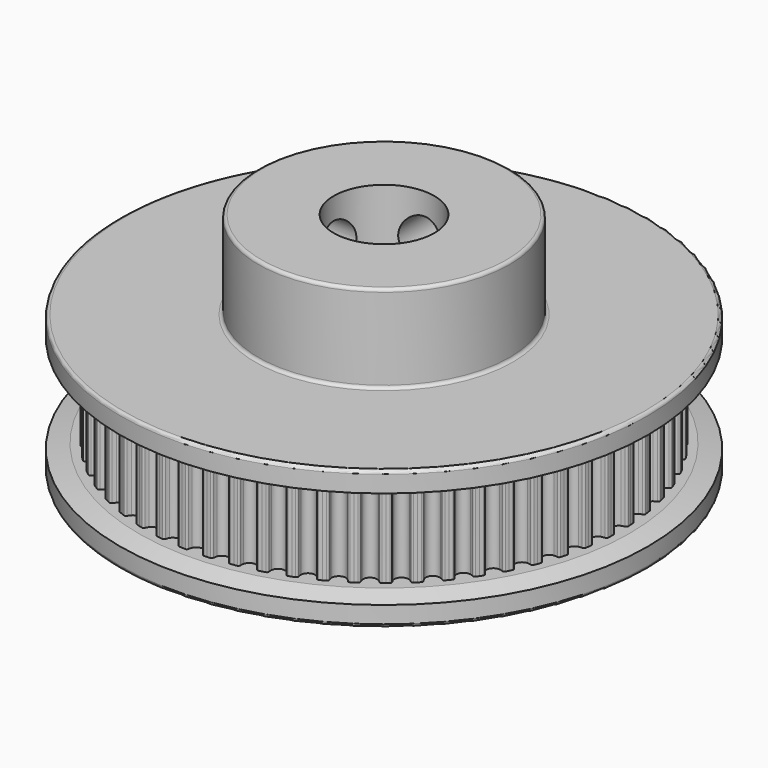
from build123d import *

# Parameters (mm, degrees)
F3_DEPTH    = 3.5
F4_COUNT    = 60
F5_R        = 21
F6_DEPTH    = 2
F7_R        = 21
F8_DEPTH    = 2
F9_R        = 10
F10_DEPTH   = 7
F11_R       = 4
F12_DEPTH   = 18.001
F13_R       = 1.75
F14_DEPTH   = 21.001
F15_R       = 1.75
F16_DEPTH   = 21.001
F17_SIZE2   = 0.4019237886
F17_SIZE    = 1.5
F17_2_SIZE2 = 0.4019237886
F17_2_SIZE  = 1.5
F18_R       = 0.25


# Not quite as in the source:
# - a feature names something its author has since deleted; it is built from what else it names


with BuildPart() as f3:
    # F2 (on Top) → F3 (new body, symmetric)
    with BuildSketch(Plane.XY):
        with BuildLine():
            ThreePointArc((0.5075672794, 18.4356928737), (0.3028425699, 18.1951004644), (0, 18.1051933345))
            ThreePointArc((0, 18.1051933345), (-0.3028425699, 18.1951004644), (-0.5075672794, 18.4356928737))
            ThreePointArc((-0.5075672794, 18.4356928737), (-0.5546426952, 18.5657821373), (-0.5833135378, 18.7011235355))
            ThreePointArc((-0.5833135378, 18.7011235355), (-0.6356764359, 18.7953689183), (-0.7377280214, 18.830147348))
            ThreePointArc((-0.7377280214, 18.830147348), (-0.8620076923, 18.8248674503), (-0.9862498036, 18.818767311))
            Line((-0.9862498036, 18.818767311), (0, 0))
            Line((0, 0), (0.9862498036, 18.818767311))
            ThreePointArc((0.9862498036, 18.818767311), (0.8620076923, 18.8248674503), (0.7377280214, 18.830147348))
            ThreePointArc((0.7377280214, 18.830147348), (0.6356764359, 18.7953689183), (0.5833135378, 18.7011235355))
            ThreePointArc((0.5833135378, 18.7011235355), (0.5546426952, 18.5657821373), (0.5075672794, 18.4356928737))
        make_face()
    extrude(amount=F3_DEPTH, both=True)

    # F4: F3 ×60 about axis
    f4_axis = Axis((0, 0, 0), (0, 0, -1))


with BuildPart() as f3_1:
    add(f3.part)
    for i in range(1, F4_COUNT):
        add(f3.part.rotate(f4_axis, i * 360 / F4_COUNT))

    # F5 (on face) → F6 (join)
    with BuildSketch(Plane(origin=(0, 0, -3.5), x_dir=(1, 0, 0), z_dir=(0, 0, -1))):
        Circle(F5_R)
    extrude(amount=F6_DEPTH)

    # F7 (on face) → F8 (join)
    with BuildSketch(Plane.XY.offset(3.5)):
        Circle(F7_R)
    extrude(amount=F8_DEPTH)

    # F9 (on face) → F10 (join)
    with BuildSketch(Plane.XY.offset(5.5)):
        Circle(F9_R)
    extrude(amount=F10_DEPTH)

    # F11 (on face) → F12 (cut, through all)
    with BuildSketch(Plane.XY.offset(12.5)):
        Circle(F11_R)
    extrude(amount=-F12_DEPTH, mode=Mode.SUBTRACT)

    # F13 (on Front) → F14 (cut, through all)
    with BuildSketch(Plane.XZ):
        with Locations((0, 9)):
            Circle(F13_R)
    extrude(amount=-F14_DEPTH, mode=Mode.SUBTRACT)

    # F15 (on Right) → F16 (cut, through all)
    with BuildSketch(Plane.YZ):
        with Locations((0, 9)):
            Circle(F15_R)
    extrude(amount=-F16_DEPTH, mode=Mode.SUBTRACT)

    # F17
    f17_edges = [f3_1.edges().sort_by_distance(p)[0] for p in [
        (-21, 0, -3.5),
    ]]
    f17_side = f3_1.faces().sort_by_distance((-20.40603, 0, -3.5))[0]
    chamfer(f17_edges, length=F17_SIZE, length2=F17_SIZE2, reference=f17_side)

    # F17#2
    f17_2_edges = [f3_1.edges().sort_by_distance(p)[0] for p in [
        (-21, 0, 3.5),
    ]]
    f17_2_side = f3_1.faces().sort_by_distance((-20.40603, 0, 3.5))[0]
    chamfer(f17_2_edges, length=F17_2_SIZE, length2=F17_2_SIZE2, reference=f17_2_side)

    # F18
    f18_edges = [f3_1.edges().sort_by_distance(p)[0] for p in [
        (-10, 0, 5.5),
        (-10, 0, 12.5),
        (-21, 0, 5.5),
        (-21, 0, -5.5),
    ]]
    fillet(f18_edges, radius=F18_R)


solid = f3_1.part
